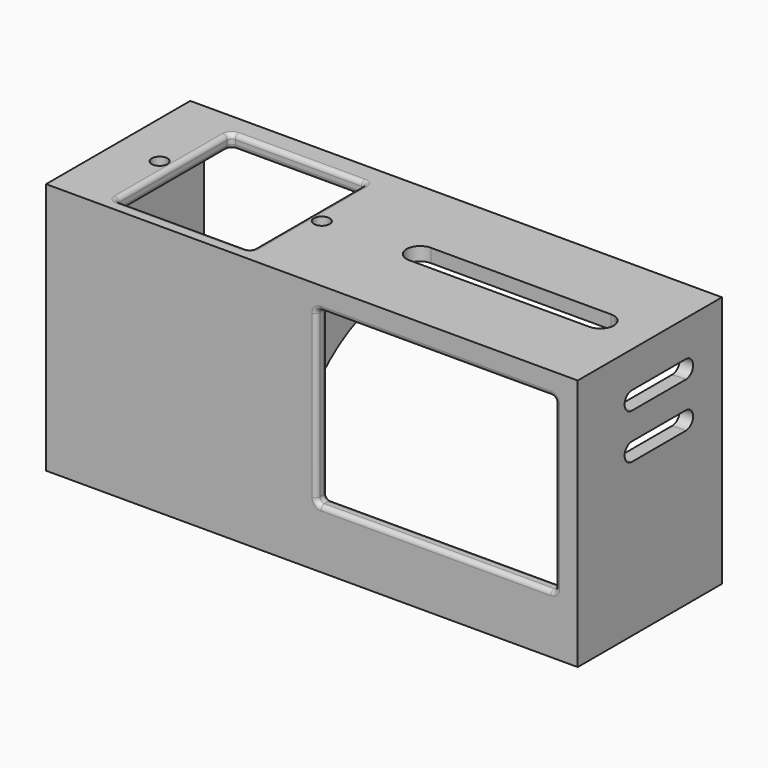
from build123d import *

# Parameters (mm, degrees)
F0_W     = 118
F0_H     = 40
F0_R     = 1.75
F0_W_2   = 30
F0_H_2   = 32
F1_DEPTH = 3
F3_DEPTH = 53
F5_DEPTH = 4
F6_W     = 53
F6_H     = 38
F7_DEPTH = 3
F9_DEPTH = 3
F10_R    = 0.99999


# Not quite as in the source:
# - a fillet or chamfer is up to 0.001 mm smaller than in the source, because OpenCascade refuses the exact size


with BuildPart() as f1:
    # F0 (on Top) → F1 (new body)
    with BuildSketch(Plane.XY):
        Rectangle(F0_W, F0_H)
        with Locations((-49, -1)):
            Circle(F0_R, mode=Mode.SUBTRACT)
        with Locations((-31, -1)):
            Rectangle(F0_W_2, F0_H_2, mode=Mode.SUBTRACT)
        with Locations((-13, -1)):
            Circle(F0_R, mode=Mode.SUBTRACT)
        with BuildLine():
            ThreePointArc((8, -3), (5, 0), (8, 3))
            Line((8, 3), (48, 3))
            ThreePointArc((48, 3), (51, 0), (48, -3))
            Line((48, -3), (8, -3))
        make_face(mode=Mode.SUBTRACT)
    extrude(amount=F1_DEPTH)

    # F2 (on face) → F3 (join)
    with BuildSketch(Plane(origin=(0, 0, 0), x_dir=(1, 0, 0), z_dir=(0, 0, -1))):
        Polygon((-56, 20), (-59, 20), (-59, 17), (-59, -20), (-56, -20), (-56, 17), (-46, 17), (-16, 17), (-6, 17), (-6, -11), (-3, -11), (-3, 17), (56, 17), (56, -20), (59, -20), (59, 17), (59, 20), (56, 20), align=None)
    extrude(amount=F3_DEPTH)

    # F4 (on face) → F5 (cut)
    with BuildSketch(Plane.YZ.offset(59)):
        with BuildLine():
            Line((10, -5), (-5, -5))
            ThreePointArc((-5, -5), (-7, -7), (-5, -9))
            Line((-5, -9), (10, -9))
            ThreePointArc((10, -9), (12, -7), (10, -5))
        make_face()
        with BuildLine():
            Line((10, -15), (-5, -15))
            ThreePointArc((-5, -15), (-7, -17), (-5, -19))
            Line((-5, -19), (10, -19))
            ThreePointArc((10, -19), (12, -17), (10, -15))
        make_face()
    extrude(amount=-F5_DEPTH, mode=Mode.SUBTRACT)

    # F6 (on face) → F7 (cut)
    with BuildSketch(Plane.XZ.offset(20)):
        with Locations((27.5, -21)):
            Rectangle(F6_W, F6_H)
    extrude(amount=-F7_DEPTH, mode=Mode.SUBTRACT)

    # F8 (on face) → F9 (cut)
    with BuildSketch(Plane.YZ.offset(-3)):
        with BuildLine():
            Line((-17, -53), (11, -53))
            Line((11, -53), (11, -23))
            Line((11, -23), (11, -10))
            ThreePointArc((11, -10), (-4.8004605743, -12.6220849169), (-17, -23))
            Line((-17, -23), (-17, -53))
        make_face()
    extrude(amount=-F9_DEPTH, mode=Mode.SUBTRACT)

    # F10 (radius 1 in the source; OpenCascade refuses exactly that, so slightly less here)
    f10_edges = [f1.edges().sort_by_distance(p)[0] for p in [
        (26.5, -17, 0),
        (-11, -17, 0),
        (-51, -17, 0),
        (27.5, -17, -2),
        (54, -20, -21),
        (27.5, -20, -40),
        (1, -20, -21),
        (1, -17, -21),
        (54, -17, -21),
        (27.5, -17, -40),
        (-16, -1, 3),
        (-31, -17, 3),
        (-46, -1, 3),
        (-31, 15, 3),
        (-31, 15, 0),
        (-16, -1, 0),
        (-46, -1, 0),
        (27.5, -20, -2),
        (-16, 15, 1.5),
        (-46, 15, 1.5),
        (-46, -17, 1.5),
        (-16, -17, 1.5),
        (54, -18.5, -2),
        (54, -18.5, -40),
        (1, -18.5, -40),
        (1, -18.5, -2),
        (-3, -3, 0),
        (-4.5, 11, 0),
        (-6, -3, 0),
        (-6, -17, -11.5),
        (-3, -17, -11.5),
        (-4.5, 11, -10),
    ]]
    fillet(f10_edges, radius=F10_R)


solid = f1.part
